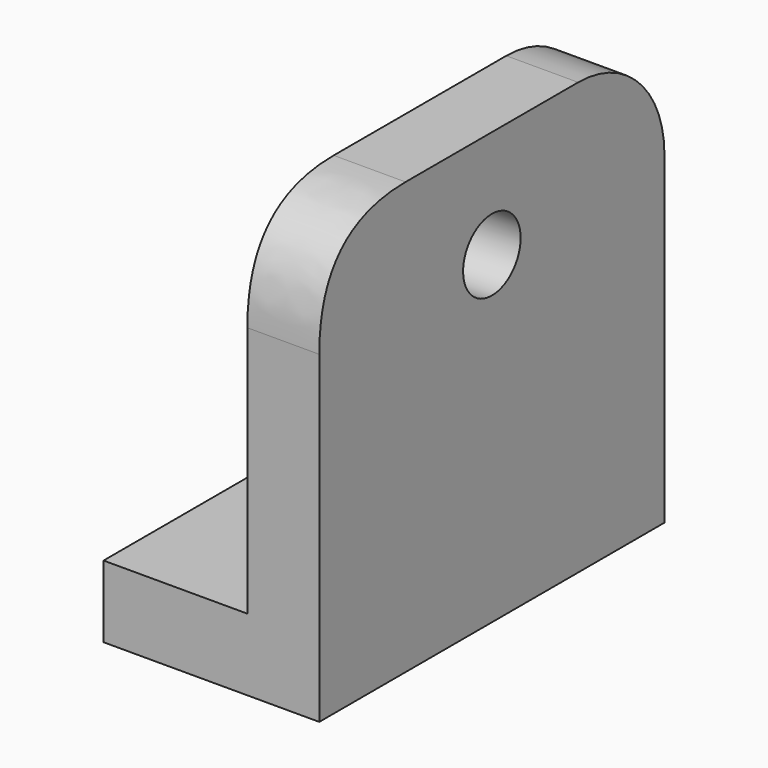
from build123d import *

# Parameters (mm, degrees)
F1_DEPTH    = 76.2
F2_R        = 12.7
F3_DEPTH    = 38.1
F5_DEPTH    = 25.4
F6_T1_DEPTH = 215.9
F7_R        = 38.1
F8_R        = 19.05
F8_R_2      = 12.7
F9_DEPTH    = 6.35


# Not quite as in the source:
# - a fillet or chamfer that OpenCascade refuses, or shapes differently, is made with other operations: its cross-section is extruded or revolved along the edge and cut away or added


with BuildPart() as f1:
    # F0 (on Front) → F1 (new body, symmetric)
    with BuildSketch(Plane.XZ):
        Polygon((-76.2, 0), (0, 0), (0, 152.4), (-25.4, 152.4), (-25.4, 25.4), (-76.2, 25.4), align=None)
    extrude(amount=F1_DEPTH, both=True)

    # F2 (on face) → F3 (cut)
    with BuildSketch(Plane.YZ):
        with Locations((0, 114.3)):
            Circle(F2_R)
    extrude(amount=-F3_DEPTH, mode=Mode.SUBTRACT)

    # F4 (on face) → F5 (cut)
    with BuildSketch(Plane.XY.offset(25.4)):
        with BuildLine():
            Line((-63.5, 12.7), (-76.2, 12.7))
            Line((-76.2, 12.7), (-76.2, -12.7))
            Line((-76.2, -12.7), (-63.5, -12.7))
            ThreePointArc((-63.5, -12.7), (-50.8, 0), (-63.5, 12.7))
        make_face()
    extrude(amount=-F5_DEPTH, mode=Mode.SUBTRACT)

    # F6: fillet of radius 38.1 on 1 edges, made by hand

    # F6_s2 → F6_t1 (cut)
    with BuildSketch(Plane.YZ.offset(-120.65)):
        with BuildLine():
            add(Edge.make_bspline(
                [(-76.2, 114.3), (-76.2, 152.4), (-38.1, 152.4)],
                knots=[0, 0, 0, 1, 1, 1], degree=2, weights=[1, 1, 1]))
            Line((-38.1, 152.4), (-76.2, 152.4))
            Line((-76.2, 152.4), (-76.2, 114.3))
        make_face()
    extrude(amount=F6_T1_DEPTH, mode=Mode.SUBTRACT)

    # F7
    f7_edges = [f1.edges().sort_by_distance(p)[0] for p in [
        (-12.7, 76.2, 152.4),
    ]]
    fillet(f7_edges, radius=F7_R)

    # F8 (on face) → F9 (cut)
    with BuildSketch(Plane(origin=(-25.4, 0, 0), x_dir=(0, -1, 0), z_dir=(-1, 0, 0))):
        with Locations((0, 114.3)):
            Circle(F8_R)
        with Locations((0, 114.3)):
            Circle(F8_R_2, mode=Mode.SUBTRACT)
    extrude(amount=-F9_DEPTH, mode=Mode.SUBTRACT)


solid = f1.part
